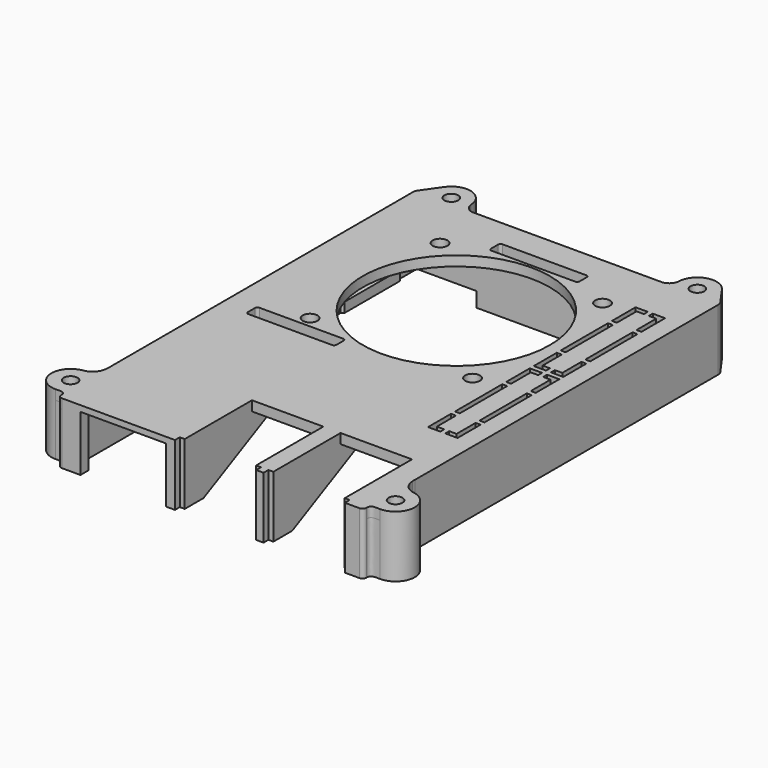
from build123d import *

# Parameters (mm, degrees)
F0_R           = 1.4
F1_DEPTH       = 2
F2_DEPTH       = 12.5
F3_R           = 1.5
F4_R           = 0.773
F5_W           = 2.8
F5_H           = 27.1
F5_W_2         = 3.5
F6_DEPTH       = 10.5
F7_SIZE2       = 10.49999
F7_SIZE        = 21.09999
F8_W           = 14.5
F8_H           = 16.3
F9_DEPTH       = 12.5
F10_W          = 17.4
F10_H          = 2
F10_H_2        = 20.7
F11_DEPTH      = 0.8
F11_DEPTH_BACK = 10.5
F13_DEPTH      = 1
F15_DEPTH      = 1
F16_W          = 21
F16_H          = 6
F17_DEPTH      = 1.5
F19_DEPTH      = 6
F20_DEPTH      = 2.4
F21_SIZE       = 0.4
F22_W          = 16.5
F22_H          = 3.9
F23_DEPTH      = 2.49
F22_W_2        = 12
F22_H_2        = 2
F24_DEPTH      = 1.5
F25_SIZE       = 0.5
F26_W          = 33.5
F26_H          = 2
F27_DEPTH      = 15.5
F28_W          = 16.5
F28_H          = 1.5
F29_DEPTH      = 1
F30_R          = 19
F30_R_2        = 1.5
F31_DEPTH      = 2
F32_W          = 1
F32_H          = 12
F32_W_2        = 18
F32_H_2        = 2.8
F33_DEPTH      = 2
F34_R          = 0.5


# Not quite as in the source:
# - a fillet or chamfer is up to 0.001 mm smaller than in the source, because OpenCascade refuses the exact size


with BuildPart() as f1:
    # F0 (on Top) → F1 (new body)
    with BuildSketch(Plane.XY):
        with BuildLine():
            Line((19.3051240806, 42.441905711), (-18.9523071583, 42.441905711))
            add(Edge.make_bspline(
                [(-18.9523071583, 42.441905711), (-19.9190404798, 42.441905711), (-20.820476913, 43.2054118672), (-20.9220278635, 44.3548110683)],
                knots=[0, 0, 0, 0, 2.7457251433, 2.7457251433, 2.7457251433, 2.7457251433], degree=3))
            ThreePointArc((-20.9220278635, 44.3548110683), (-23.7216768108, 47.9310673065), (-28.0087973477, 46.4316539507))
            Line((-28.0087973477, 46.4316539507), (-30.8140766407, 42.441905711))
            Line((-30.8140766407, 42.441905711), (-30.8140766407, -34.9979682407))
            add(Edge.make_bspline(
                [(-30.8140766407, -34.9979682407), (-30.7986160442, -35.2346444142), (-30.799145406, -35.4584579304), (-30.8140766407, -35.6697973339)],
                knots=[0, 0, 0, 0, 0.4551566215, 0.4551566215, 0.4551566215, 0.4551566215], degree=3))
            add(Edge.make_bspline(
                [(-30.8140766407, -35.6697973339), (-30.9484119796, -37.5712040795), (-32.2485044438, -38.462895914), (-33.5578223104, -38.6278325259)],
                knots=[0.4551566215, 0.4551566215, 0.4551566215, 0.4551566215, 4.5501708791, 4.5501708791, 4.5501708791, 4.5501708791], degree=3))
            ThreePointArc((-33.5578223104, -38.6278325259), (-36.7050696781, -42.8377355072), (-32.8017436583, -46.3580330924))
            add(Edge.make_bspline(
                [(-30.8140766407, -47.4269150338), (-30.8531735624, -46.2938717148), (-31.3508648957, -46.3264760931), (-32.8017436583, -46.3580330924)],
                knots=[0, 0, 0, 0, 2.2568404412, 2.2568404412, 2.2568404412, 2.2568404412], degree=3))
            Line((-30.8140766407, -47.4269150338), (-30.8140766407, -48.158094289))
            Line((-30.8140766407, -48.158094289), (31.1859233593, -48.158094289))
            Line((31.1859233593, -48.158094289), (31.1859233593, -47.1719584179))
            add(Edge.make_bspline(
                [(31.1859233593, -47.1719584179), (31.2936567608, -46.2991912107), (31.8221947799, -46.3290537815), (33.1545605807, -46.3580330924)],
                knots=[0.1843467916, 0.1843467916, 0.1843467916, 0.1843467916, 2.2568404412, 2.2568404412, 2.2568404412, 2.2568404412], degree=3))
            ThreePointArc((33.1545605807, -46.3580330924), (37.0578866004, -42.8377355072), (33.9106392328, -38.6278325259))
            add(Edge.make_bspline(
                [(31.1859233593, -35.677425735), (31.3200805447, -37.573589439), (32.6030735958, -38.4631166448), (33.9106392328, -38.6278325259)],
                knots=[0.4594777879, 0.4594777879, 0.4594777879, 0.4594777879, 4.5387213301, 4.5387213301, 4.5387213301, 4.5387213301], degree=3))
            add(Edge.make_bspline(
                [(31.1859233605, -34.9979682409), (31.1702766124, -35.2374940874), (31.1708121637, -35.4638456691), (31.1859233593, -35.677425735)],
                knots=[0, 0, 0, 0, 0.4594777879, 0.4594777879, 0.4594777879, 0.4594777879], degree=3))
            Line((31.1859233593, -34.9979682409), (31.1859233593, 42.441905711))
            Line((31.1859233593, 42.441905711), (28.3616142701, 46.4316539507))
            ThreePointArc((28.3616142701, 46.4316539507), (24.0744937332, 47.9310673065), (21.2748447859, 44.3548110683))
            add(Edge.make_bspline(
                [(19.3051240806, 42.441905711), (20.2718574022, 42.441905711), (21.1732938354, 43.2054118672), (21.2748447859, 44.3548110683)],
                knots=[0, 0, 0, 0, 2.7457251433, 2.7457251433, 2.7457251433, 2.7457251433], degree=3))
        make_face()
        with Locations((-32.8235915388, -42.458094289)):
            Circle(F0_R, mode=Mode.SUBTRACT)
        with Locations((33.1764084612, -42.458094289)):
            Circle(F0_R, mode=Mode.SUBTRACT)
        with BuildLine():
            Line((28.6859233593, -46.158094289), (-28.3140766407, -46.158094289))
            ThreePointArc((-28.3140766407, -46.158094289), (-28.6676300313, -46.0116476796), (-28.8140766407, -45.658094289))
            Line((-28.8140766407, -45.658094289), (-28.8140766407, 39.941905711))
            ThreePointArc((-28.8140766407, 39.941905711), (-28.6676300313, 40.2954591016), (-28.3140766407, 40.441905711))
            Line((-28.3140766407, 40.441905711), (28.6859233593, 40.441905711))
            ThreePointArc((28.6859233593, 40.441905711), (29.0394767498, 40.2954591016), (29.1859233593, 39.941905711))
            Line((29.1859233593, 39.941905711), (29.1859233593, -45.658094289))
            ThreePointArc((29.1859233593, -45.658094289), (29.0394767498, -46.0116476796), (28.6859233593, -46.158094289))
        make_face(mode=Mode.SUBTRACT)
        with Locations((-24.8184789504, 44.1884712735)):
            Circle(F0_R, mode=Mode.SUBTRACT)
        with Locations((25.1712958728, 44.1884712735)):
            Circle(F0_R, mode=Mode.SUBTRACT)
        with BuildLine():
            ThreePointArc((-28.8140766407, -45.658094289), (-28.6676300313, -46.0116476796), (-28.3140766407, -46.158094289))
            Line((-28.3140766407, -46.158094289), (28.6859233593, -46.158094289))
            ThreePointArc((28.6859233593, -46.158094289), (29.0394767498, -46.0116476796), (29.1859233593, -45.658094289))
            Line((29.1859233593, -45.658094289), (29.1859233593, 39.941905711))
            ThreePointArc((29.1859233593, 39.941905711), (29.0394767498, 40.2954591016), (28.6859233593, 40.441905711))
            Line((28.6859233593, 40.441905711), (-28.3140766407, 40.441905711))
            ThreePointArc((-28.3140766407, 40.441905711), (-28.6676300313, 40.2954591016), (-28.8140766407, 39.941905711))
            Line((-28.8140766407, 39.941905711), (-28.8140766407, -45.658094289))
        make_face()
    extrude(amount=-F1_DEPTH)

    # F0 (on Top) → F2 (join)
    with BuildSketch(Plane.XY):
        with BuildLine():
            Line((19.3051240806, 42.441905711), (-18.9523071583, 42.441905711))
            add(Edge.make_bspline(
                [(-18.9523071583, 42.441905711), (-19.9190404798, 42.441905711), (-20.820476913, 43.2054118672), (-20.9220278635, 44.3548110683)],
                knots=[0, 0, 0, 0, 2.7457251433, 2.7457251433, 2.7457251433, 2.7457251433], degree=3))
            ThreePointArc((-20.9220278635, 44.3548110683), (-23.7216768108, 47.9310673065), (-28.0087973477, 46.4316539507))
            Line((-28.0087973477, 46.4316539507), (-30.8140766407, 42.441905711))
            Line((-30.8140766407, 42.441905711), (-30.8140766407, -34.9979682407))
            add(Edge.make_bspline(
                [(-30.8140766407, -34.9979682407), (-30.7986160442, -35.2346444142), (-30.799145406, -35.4584579304), (-30.8140766407, -35.6697973339)],
                knots=[0, 0, 0, 0, 0.4551566215, 0.4551566215, 0.4551566215, 0.4551566215], degree=3))
            add(Edge.make_bspline(
                [(-30.8140766407, -35.6697973339), (-30.9484119796, -37.5712040795), (-32.2485044438, -38.462895914), (-33.5578223104, -38.6278325259)],
                knots=[0.4551566215, 0.4551566215, 0.4551566215, 0.4551566215, 4.5501708791, 4.5501708791, 4.5501708791, 4.5501708791], degree=3))
            ThreePointArc((-33.5578223104, -38.6278325259), (-36.7050696781, -42.8377355072), (-32.8017436583, -46.3580330924))
            add(Edge.make_bspline(
                [(-30.8140766407, -47.4269150338), (-30.8531735624, -46.2938717148), (-31.3508648957, -46.3264760931), (-32.8017436583, -46.3580330924)],
                knots=[0, 0, 0, 0, 2.2568404412, 2.2568404412, 2.2568404412, 2.2568404412], degree=3))
            Line((-30.8140766407, -47.4269150338), (-30.8140766407, -48.158094289))
            Line((-30.8140766407, -48.158094289), (31.1859233593, -48.158094289))
            Line((31.1859233593, -48.158094289), (31.1859233593, -47.1719584179))
            add(Edge.make_bspline(
                [(31.1859233593, -47.1719584179), (31.2936567608, -46.2991912107), (31.8221947799, -46.3290537815), (33.1545605807, -46.3580330924)],
                knots=[0.1843467916, 0.1843467916, 0.1843467916, 0.1843467916, 2.2568404412, 2.2568404412, 2.2568404412, 2.2568404412], degree=3))
            ThreePointArc((33.1545605807, -46.3580330924), (37.0578866004, -42.8377355072), (33.9106392328, -38.6278325259))
            add(Edge.make_bspline(
                [(31.1859233593, -35.677425735), (31.3200805447, -37.573589439), (32.6030735958, -38.4631166448), (33.9106392328, -38.6278325259)],
                knots=[0.4594777879, 0.4594777879, 0.4594777879, 0.4594777879, 4.5387213301, 4.5387213301, 4.5387213301, 4.5387213301], degree=3))
            add(Edge.make_bspline(
                [(31.1859233605, -34.9979682409), (31.1702766124, -35.2374940874), (31.1708121637, -35.4638456691), (31.1859233593, -35.677425735)],
                knots=[0, 0, 0, 0, 0.4594777879, 0.4594777879, 0.4594777879, 0.4594777879], degree=3))
            Line((31.1859233593, -34.9979682409), (31.1859233593, 42.441905711))
            Line((31.1859233593, 42.441905711), (28.3616142701, 46.4316539507))
            ThreePointArc((28.3616142701, 46.4316539507), (24.0744937332, 47.9310673065), (21.2748447859, 44.3548110683))
            add(Edge.make_bspline(
                [(19.3051240806, 42.441905711), (20.2718574022, 42.441905711), (21.1732938354, 43.2054118672), (21.2748447859, 44.3548110683)],
                knots=[0, 0, 0, 0, 2.7457251433, 2.7457251433, 2.7457251433, 2.7457251433], degree=3))
        make_face()
        with Locations((-32.8235915388, -42.458094289)):
            Circle(F0_R, mode=Mode.SUBTRACT)
        with Locations((33.1764084612, -42.458094289)):
            Circle(F0_R, mode=Mode.SUBTRACT)
        with BuildLine():
            Line((28.6859233593, -46.158094289), (-28.3140766407, -46.158094289))
            ThreePointArc((-28.3140766407, -46.158094289), (-28.6676300313, -46.0116476796), (-28.8140766407, -45.658094289))
            Line((-28.8140766407, -45.658094289), (-28.8140766407, 39.941905711))
            ThreePointArc((-28.8140766407, 39.941905711), (-28.6676300313, 40.2954591016), (-28.3140766407, 40.441905711))
            Line((-28.3140766407, 40.441905711), (28.6859233593, 40.441905711))
            ThreePointArc((28.6859233593, 40.441905711), (29.0394767498, 40.2954591016), (29.1859233593, 39.941905711))
            Line((29.1859233593, 39.941905711), (29.1859233593, -45.658094289))
            ThreePointArc((29.1859233593, -45.658094289), (29.0394767498, -46.0116476796), (28.6859233593, -46.158094289))
        make_face(mode=Mode.SUBTRACT)
        with Locations((-24.8184789504, 44.1884712735)):
            Circle(F0_R, mode=Mode.SUBTRACT)
        with Locations((25.1712958728, 44.1884712735)):
            Circle(F0_R, mode=Mode.SUBTRACT)
    extrude(amount=-F2_DEPTH)

    # F3
    f3_edges = [f1.edges().sort_by_distance(p)[0] for p in [
        (-30.814077, 42.441906, -6.25),
        (31.185923, 42.441906, -6.25),
    ]]
    fillet(f3_edges, radius=F3_R)

    # F4
    f4_edges = [f1.edges().sort_by_distance(p)[0] for p in [
        (-30.814077, -48.158094, -6.25),
        (31.185923, -48.158094, -6.25),
    ]]
    fillet(f4_edges, radius=F4_R)

    # F5 (on face) → F6 (join)
    with BuildSketch(Plane(origin=(0, 0, -2), x_dir=(1, 0, 0), z_dir=(0, 0, -1))):
        with Locations((-7.474, 34.608094289)):
            Rectangle(F5_W, F5_H)
        with Locations((10.176, 34.608094289)):
            Rectangle(F5_W_2, F5_H)
    extrude(amount=F6_DEPTH)

    # F7 (size 21.1 and 10.5 in the source; OpenCascade refuses exactly that, so slightly less here)
    f7_edges = [f1.edges().sort_by_distance(p)[0] for p in [
        (-7.474, -21.058094, -12.5),
        (10.176, -21.058094, -12.5),
    ]]
    f7_side = f1.faces().sort_by_distance((-31.218411, -45.211298, -12.5))[0]
    chamfer(f7_edges, length=F7_SIZE, length2=F7_SIZE2, reference=f7_side)

    # F8 (on face) → F9 (cut, through all)
    with BuildSketch(Plane.XY):
        Polygon((8.426, -46.158094289), (-6.074, -46.158094289), (-6.074, -46.928094289), (-7.074, -46.928094289), (-7.074, -48.158094289), (-6.074, -48.158094289), (8.426, -48.158094289), (9.426, -48.158094289), (9.426, -46.928094289), (8.426, -46.928094289), align=None)
        with Locations((1.176, -38.008094289)):
            Rectangle(F8_W, F8_H)
        Polygon((26.426, -46.158094289), (11.926, -46.158094289), (11.926, -46.928094289), (10.926, -46.928094289), (10.926, -48.158094289), (11.926, -48.158094289), (26.426, -48.158094289), (27.426, -48.158094289), (27.426, -46.928094289), (26.426, -46.928094289), align=None)
        with Locations((19.176, -38.008094289)):
            Rectangle(F8_W, F8_H)
    extrude(amount=-F9_DEPTH, mode=Mode.SUBTRACT)

    # F10 (on face) → F11 (cut, two sides)
    with BuildSketch(Plane(origin=(0, 0, -2), x_dir=(1, 0, 0), z_dir=(0, 0, -1))) as f11_sk:
        with Locations((-17.574, 47.158094289)):
            Rectangle(F10_W, F10_H)
        with Locations((-17.574, 35.808094289)):
            Rectangle(F10_W, F10_H_2)
    extrude(amount=-F11_DEPTH, mode=Mode.SUBTRACT)
    extrude(f11_sk.sketch, amount=F11_DEPTH_BACK, mode=Mode.SUBTRACT)

    # F12 (on face) → F13 (cut)
    with BuildSketch(Plane(origin=(-30.8140766407, 0, 0), x_dir=(0, -1, 0), z_dir=(-1, 0, 0))):
        with BuildLine():
            Line((9.7100105214, -12.5), (19.2099894786, -12.5))
            ThreePointArc((19.2099894786, -12.5), (14.46, -7.7599976439), (9.7100105214, -12.5))
        make_face()
    extrude(amount=-F13_DEPTH, mode=Mode.SUBTRACT)

    # F14 (on face) → F15 (cut, through all)
    with BuildSketch(Plane(origin=(-29.8140766407, 0, 0), x_dir=(0, -1, 0), z_dir=(-1, 0, 0))):
        with BuildLine():
            Line((10.960014279, -12.5), (17.959985721, -12.5))
            ThreePointArc((17.959985721, -12.5), (14.46, -9.0099976439), (10.960014279, -12.5))
        make_face()
    extrude(amount=-F15_DEPTH, mode=Mode.SUBTRACT)

    # F16 (on face) → F17 (cut)
    with BuildSketch(Plane(origin=(-30.8140766407, 0, 0), x_dir=(0, -1, 0), z_dir=(-1, 0, 0))):
        with Locations((-7.0899894786, -9.5)):
            Rectangle(F16_W, F16_H)
    extrude(amount=-F17_DEPTH, mode=Mode.SUBTRACT)

    # F18 (on face) → F19 (join)
    with BuildSketch(Plane(origin=(0, 0, -12.5), x_dir=(1, 0, 0), z_dir=(0, 0, -1))):
        Polygon((-28.3240766407, 4.408094289), (-28.8140766407, 4.898094289), (-28.8140766407, -19.101905711), (-28.3240766407, -18.611905711), align=None)
    extrude(amount=-F19_DEPTH)

    # F18 (on face) → F20 (join)
    with BuildSketch(Plane(origin=(0, 0, -12.5), x_dir=(1, 0, 0), z_dir=(0, 0, -1))):
        Polygon((-28.3240766407, 4.408094289), (-28.8140766407, 4.898094289), (-28.8140766407, -19.101905711), (-28.3240766407, -18.611905711), align=None)
        Polygon((-28.3240766407, -21.501905711), (-28.8140766407, -21.011905711), (-28.8140766407, -36.011905711), (-28.3240766407, -35.521905711), align=None)
    extrude(amount=-F20_DEPTH)

    # F21
    f21_edges = [f1.edges().sort_by_distance(p)[0] for p in [
        (-28.324077, 28.511906, -10.1),
        (-28.324077, 7.101906, -6.5),
    ]]
    chamfer(f21_edges, length=F21_SIZE)

    # F22 (on face) → F23 (cut, through all)
    with BuildSketch(Plane(origin=(-30.8140766407, 0, 0), x_dir=(0, -1, 0), z_dir=(-1, 0, 0))):
        with Locations((-7.1212481916, -10.55)):
            Rectangle(F22_W, F22_H)
    extrude(amount=-F23_DEPTH, mode=Mode.SUBTRACT)

    # F22 (on face) → F24 (cut)
    with BuildSketch(Plane(origin=(-30.8140766407, 0, 0), x_dir=(0, -1, 0), z_dir=(-1, 0, 0))):
        with Locations((-28.5212481916, -11.5)):
            Rectangle(F22_W_2, F22_H_2)
    extrude(amount=-F24_DEPTH, mode=Mode.SUBTRACT)

    # F25
    f25_edges = [f1.edges().sort_by_distance(p)[0] for p in [
        (-29.314077, 17.589989, -9.5),
        (-29.314077, 7.089989, -6.5),
        (-29.314077, -3.410011, -9.5),
        (-29.314077, 34.521248, -11.5),
        (-29.314077, 28.521248, -10.5),
        (-29.314077, 22.521248, -11.5),
    ]]
    chamfer(f25_edges, length=F25_SIZE)

    # F26 (on Top) → F27 (join)
    with BuildSketch(Plane.XY):
        with Locations((0.1, 41.441905711)):
            Rectangle(F26_W, F26_H)
    extrude(amount=-F27_DEPTH)

    # F28 (on face) → F29 (cut)
    with BuildSketch(Plane(origin=(0, 42.441905711, 0), x_dir=(-1, 0, 0), z_dir=(0, 1, 0))):
        with Locations((-0.176, -14.75)):
            Rectangle(F28_W, F28_H)
    extrude(amount=-F29_DEPTH, mode=Mode.SUBTRACT)

    # F30 (on face) → F31 (cut, through all)
    with BuildSketch(Plane.XY):
        with Locations((0, 14.441905711)):
            Circle(F30_R)
        with Locations((-16.5, 30.941905711)):
            Circle(F30_R_2)
        with Locations((-16.5, -2.058094289)):
            Circle(F30_R_2)
        with Locations((16.5, 30.941905711)):
            Circle(F30_R_2)
        with Locations((16.5, -2.058094289)):
            Circle(F30_R_2)
    extrude(amount=-F31_DEPTH, mode=Mode.SUBTRACT)

    # F32 (on face) → F33 (cut, through all)
    with BuildSketch(Plane.XY):
        Polygon((22.4859233593, 27.091905711), (22.4859233593, 32.091905711), (23.9859233593, 32.091905711), (23.9859233593, 33.091905711), (21.4859233593, 33.091905711), (21.4859233593, 27.091905711), align=None)
        Polygon((24.9859233593, 33.091905711), (24.9859233593, 32.091905711), (26.4859233593, 32.091905711), (26.4859233593, 27.091905711), (27.4859233593, 27.091905711), (27.4859233593, 33.091905711), align=None)
        with Locations((21.9859233593, 20.091905711)):
            Rectangle(F32_W, F32_H)
        with Locations((26.9859233593, 20.091905711)):
            Rectangle(F32_W, F32_H)
        Polygon((22.4859233593, 8.241905711), (22.4859233593, 13.091905711), (21.4859233593, 13.091905711), (21.4859233593, 7.241905711), (23.9859233593, 7.241905711), (23.9859233593, 8.241905711), align=None)
        Polygon((27.4859233593, 13.091905711), (26.4859233593, 13.091905711), (26.4859233593, 8.241905711), (24.9859233593, 8.241905711), (24.9859233593, 7.241905711), (27.4859233593, 7.241905711), align=None)
        Polygon((22.4859233593, 0.241905711), (22.4859233593, 5.241905711), (23.9859233593, 5.241905711), (23.9859233593, 6.241905711), (21.4859233593, 6.241905711), (21.4859233593, 0.241905711), align=None)
        Polygon((24.9859233593, 6.241905711), (24.9859233593, 5.241905711), (26.4859233593, 5.241905711), (26.4859233593, 0.241905711), (27.4859233593, 0.241905711), (27.4859233593, 6.241905711), align=None)
        with Locations((21.9859233593, -6.758094289)):
            Rectangle(F32_W, F32_H)
        with Locations((26.9859233593, -6.758094289)):
            Rectangle(F32_W, F32_H)
        Polygon((22.4859233593, -18.608094289), (22.4859233593, -13.758094289), (21.4859233593, -13.758094289), (21.4859233593, -19.608094289), (23.9859233593, -19.608094289), (23.9859233593, -18.608094289), align=None)
        Polygon((27.4859233593, -13.758094289), (26.4859233593, -13.758094289), (26.4859233593, -18.608094289), (24.9859233593, -18.608094289), (24.9859233593, -19.608094289), (27.4859233593, -19.608094289), align=None)
        with Locations((-16.5, -5.7)):
            Rectangle(F32_W_2, F32_H_2)
        with Locations((0, 35.4)):
            Rectangle(F32_W_2, F32_H_2)
    extrude(amount=-F33_DEPTH, mode=Mode.SUBTRACT)

    # F34
    f34_edges = [f1.edges().sort_by_distance(p)[0] for p in [
        (-25.5, -4.3, -1),
        (-25.5, -7.1, -1),
        (-7.5, -7.1, -1),
        (-7.5, -4.3, -1),
        (9, 36.8, -1),
        (-9, 36.8, -1),
        (-9, 34, -1),
        (9, 34, -1),
    ]]
    fillet(f34_edges, radius=F34_R)


solid = f1.part
